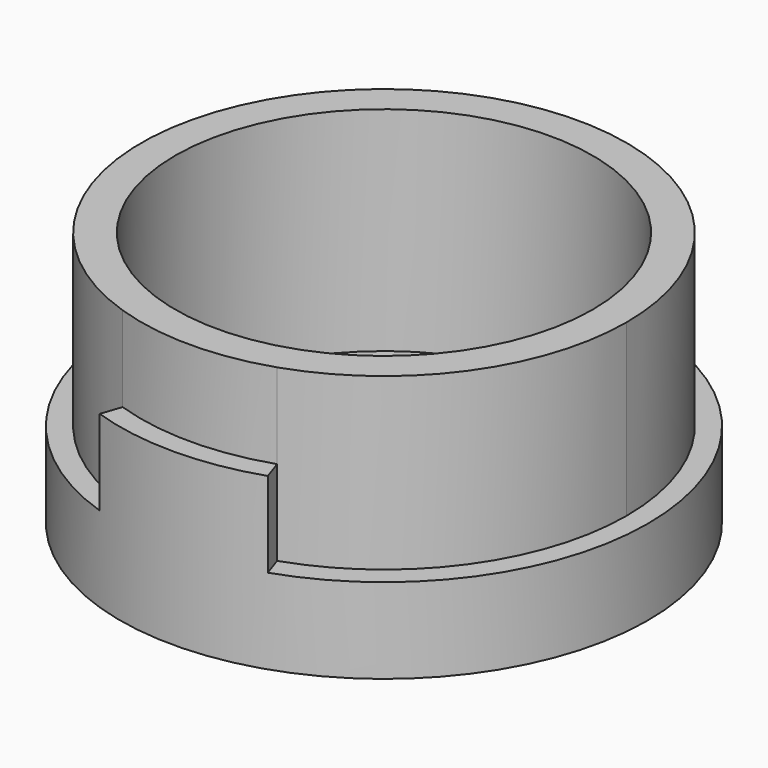
from build123d import *
from build123d import SkipClean  # not in build123d's __all__

# Parameters (mm, degrees)
F1_DEPTH = 10
F0_R     = 24.5
F2_DEPTH = 30
F3_DEPTH = 20
F4_DEPTH = 20
F5_DEPTH = 30
F6_DEPTH = 5


with BuildPart() as f1:
    # F0 (on Top) → F1 (new body)
    with BuildSketch(Plane.XY):
        with BuildLine():
            ThreePointArc((-9.06851449, 27.018735073), (0, 28.5), (9.06851449, 27.018735073))
            Line((9.06851449, 27.018735073), (9.8690700263, 29.3870967742))
            ThreePointArc((9.8690700263, 29.3870967742), (0, 31), (-9.8690700263, 29.3870967742))
            Line((-9.8690700263, 29.3870967742), (-9.06851449, 27.018735073))
        make_face()
        with BuildLine():
            ThreePointArc((-9.06851449, -27.018735073), (-28.5, 0), (-9.06851449, 27.018735073))
            Line((-9.06851449, 27.018735073), (-9.8690700263, 29.3870967742))
            ThreePointArc((-9.8690700263, 29.3870967742), (-31, 0), (-9.8690700263, -29.3870967742))
            Line((-9.8690700263, -29.3870967742), (-9.06851449, -27.018735073))
        make_face()
        with BuildLine():
            Line((9.8690700263, -29.3870967742), (9.06851449, -27.018735073))
            ThreePointArc((9.06851449, -27.018735073), (0, -28.5), (-9.06851449, -27.018735073))
            Line((-9.06851449, -27.018735073), (-9.8690700263, -29.3870967742))
            ThreePointArc((-9.8690700263, -29.3870967742), (0, -31), (9.8690700263, -29.3870967742))
        make_face()
        with BuildLine():
            ThreePointArc((9.06851449, 27.018735073), (23.1376604583, 16.6402724893), (28.5, 0))
            ThreePointArc((28.5, 0), (23.1376604583, -16.6402724893), (9.06851449, -27.018735073))
            Line((9.06851449, -27.018735073), (9.8690700263, -29.3870967742))
            ThreePointArc((9.8690700263, -29.3870967742), (25.1688415587, -18.0977737469), (31, 0))
            ThreePointArc((31, 0), (25.1688415587, 18.0977737469), (9.8690700263, 29.3870967742))
            Line((9.8690700263, 29.3870967742), (9.06851449, 27.018735073))
        make_face()
    extrude(amount=F1_DEPTH)

    # F0 (on Top) → F2 (cut)
    with BuildSketch(Plane.XY):
        with BuildLine():
            ThreePointArc((9.06851449, -27.018735073), (23.1376604583, -16.6402724893), (28.5, 0))
            ThreePointArc((28.5, 0), (23.1376604583, 16.6402724893), (9.06851449, 27.018735073))
            ThreePointArc((9.06851449, 27.018735073), (0, 28.5), (-9.06851449, 27.018735073))
            ThreePointArc((-9.06851449, 27.018735073), (-28.5, 0), (-9.06851449, -27.018735073))
            ThreePointArc((-9.06851449, -27.018735073), (0, -28.5), (9.06851449, -27.018735073))
        make_face()
        Circle(F0_R, mode=Mode.SUBTRACT)
    extrude(amount=F2_DEPTH, mode=Mode.SUBTRACT)

    # F0 (on Top) → F3 (join)
    with BuildSketch(Plane.XY):
        with BuildLine():
            ThreePointArc((-9.06851449, 27.018735073), (0, 28.5), (9.06851449, 27.018735073))
            Line((9.06851449, 27.018735073), (9.8690700263, 29.3870967742))
            ThreePointArc((9.8690700263, 29.3870967742), (0, 31), (-9.8690700263, 29.3870967742))
            Line((-9.8690700263, 29.3870967742), (-9.06851449, 27.018735073))
        make_face()
    with SkipClean():  # cleaning this boolean's faces spoils the solid; the shape is the same uncleaned
        extrude(amount=F3_DEPTH)

    # F0 (on Top) → F4 (join)
    with BuildSketch(Plane.XY):
        with BuildLine():
            Line((9.8690700263, -29.3870967742), (9.06851449, -27.018735073))
            ThreePointArc((9.06851449, -27.018735073), (0, -28.5), (-9.06851449, -27.018735073))
            Line((-9.06851449, -27.018735073), (-9.8690700263, -29.3870967742))
            ThreePointArc((-9.8690700263, -29.3870967742), (0, -31), (9.8690700263, -29.3870967742))
        make_face()
    with SkipClean():  # cleaning this boolean's faces spoils the solid; the shape is the same uncleaned
        extrude(amount=F4_DEPTH)

    # F0 (on Top) → F5 (join)
    with BuildSketch(Plane.XY):
        with BuildLine():
            ThreePointArc((9.06851449, -27.018735073), (23.1376604583, -16.6402724893), (28.5, 0))
            ThreePointArc((28.5, 0), (23.1376604583, 16.6402724893), (9.06851449, 27.018735073))
            ThreePointArc((9.06851449, 27.018735073), (0, 28.5), (-9.06851449, 27.018735073))
            ThreePointArc((-9.06851449, 27.018735073), (-28.5, 0), (-9.06851449, -27.018735073))
            ThreePointArc((-9.06851449, -27.018735073), (0, -28.5), (9.06851449, -27.018735073))
        make_face()
        Circle(F0_R, mode=Mode.SUBTRACT)
    extrude(amount=F5_DEPTH)

    # F0 (on Top) → F6 (join)
    with BuildSketch(Plane.XY):
        Circle(F0_R)
    extrude(amount=F6_DEPTH)


solid = f1.part
